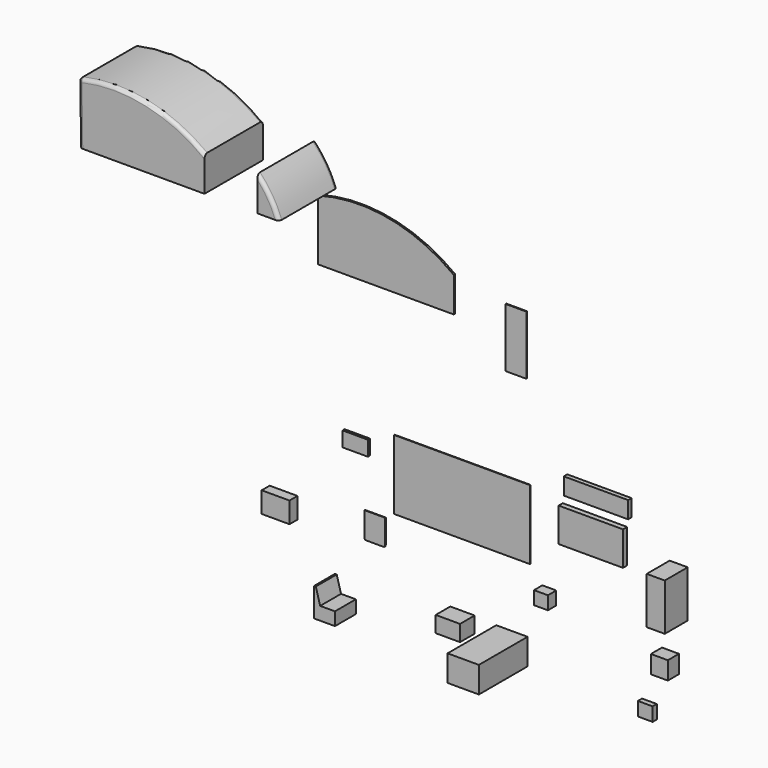
from build123d import *

# Parameters (mm, degrees)
F0_W      = 3962.4
F0_H      = 2032
F1_DEPTH  = 19.05
F0_W_2    = 527.05
F0_H_2    = 1371.6
F2_DEPTH  = 838.2
F0_W_3    = 495.3
F0_H_3    = 523.875
F3_DEPTH  = 406.4
F0_W_4    = 429.768
F0_H_4    = 400.05
F4_DEPTH  = 152.4
F0_W_5    = 741.68
F0_H_5    = 436.88
F5_DEPTH  = 76.2
F6_DEPTH  = 50.8
F7_DEPTH  = 19.05
F8_DEPTH  = 762
F9_DEPTH  = 2133.6
F0_W_6    = 609.6
F0_H_6    = 1727.2
F10_DEPTH = 25.4
F0_W_7    = 406.4
F0_H_7    = 387.35
F11_DEPTH = 304.8
F0_W_8    = 914.4
F0_H_8    = 762
F12_DEPTH = 1778
F0_W_9    = 711.2
F0_H_9    = 469.9
F13_DEPTH = 533.4
F14_DEPTH = 2133.6
F15_R     = 105.4762589975
F16_R     = 101.6
F16_2_R   = 101.6
F0_W_10   = 1879.6
F0_H_10   = 990.6
F17_DEPTH = 152.4
F18_DEPTH = 292.1
F0_H_11   = 495.3
F19_DEPTH = 127


# Not quite as in the source:
# - ends of sketch curves that miss each other by under 0.0002 mm in the source are joined


with BuildPart() as f1:
    # F0 (on Front) → F1 (new body)
    with BuildSketch(Plane.XZ):
        with Locations((-1277.7160794973, 1919.1620025635)):
            Rectangle(F0_W, F0_H)
    extrude(amount=F1_DEPTH)


with BuildPart() as f2:
    # F0 (on Front) → F2 (new body)
    with BuildSketch(Plane.XZ):
        with Locations((5036.8647483826, 1623.0339844704)):
            Rectangle(F0_W_2, F0_H_2)
    extrude(amount=F2_DEPTH)


with BuildPart() as f3:
    # F0 (on Front) → F3 (new body)
    with BuildSketch(Plane.XZ):
        with Locations((4797.2844566345, -261.9375)):
            Rectangle(F0_W_3, F0_H_3)
    extrude(amount=F3_DEPTH)


with BuildPart() as f4:
    # F0 (on Front) → F4 (new body)
    with BuildSketch(Plane.XZ):
        with Locations((4182.0682132568, -1700.6525627136)):
            Rectangle(F0_W_4, F0_H_4)
    extrude(amount=F4_DEPTH)


with BuildPart() as f5:
    # F0 (on Front) → F5 (new body)
    with BuildSketch(Plane.XZ):
        with Locations((-4351.5760449982, 2382.3956884766)):
            Rectangle(F0_W_5, F0_H_5)
    extrude(amount=F5_DEPTH)


with BuildPart() as f6:
    # F0 (on Front) → F6 (new body)
    with BuildSketch(Plane.XZ):
        with BuildLine():
            Line((-5455.5745124817, 8393.684387207), (-5455.5745124817, 6621.967618318))
            Line((-5455.5745124817, 6621.967618318), (-1493.1745124817, 6621.967618318))
            Line((-1493.1745124817, 6621.967618318), (-1493.1745124817, 7637.967618318))
            ThreePointArc((-1493.1745124817, 7637.967618318), (-3386.1147979663, 8478.5923554399), (-5455.5745124817, 8393.684387207))
        make_face()
    extrude(amount=F6_DEPTH)


with BuildPart() as f7:
    # F0 (on Front) → F7 (new body)
    with BuildSketch(Plane.XZ):
        with BuildLine():
            Line((-3521.931886673, 719.1577055931), (-4131.531886673, 719.1577055931))
            Line((-4131.531886673, 719.1577055931), (-4131.531886673, 7.9577055931))
            ThreePointArc((-4131.531886673, 7.9577055931), (-4116.6529111573, -27.9633188912), (-4080.731886673, -42.8422944069))
            Line((-4080.731886673, -42.8422944069), (-3572.731886673, -42.8422944069))
            ThreePointArc((-3572.731886673, -42.8422944069), (-3536.8108621887, -27.9633188912), (-3521.931886673, 7.9577055931))
            Line((-3521.931886673, 7.9577055931), (-3521.931886673, 719.1577055931))
        make_face()
    extrude(amount=F7_DEPTH)


with BuildPart() as f8:
    # F0 (on Front) → F8 (new body)
    with BuildSketch(Plane.XZ):
        Polygon((-4828.4018974304, -1668.460726738), (-4955.4018974304, -1211.260726738), (-5006.2018974304, -1211.260726738), (-5006.2018974304, -2049.460726738), (-4955.4018974304, -2049.460726738), (-4396.6018974304, -2049.460726738), (-4396.6018974304, -1668.460726738), align=None)
    extrude(amount=F8_DEPTH)


with BuildPart() as f9:
    # F0 (on Front) → F9 (new body)
    with BuildSketch(Plane.XZ):
        with BuildLine():
            Line((-10793.848991394, 10522.1261978149), (-10768.254913326, 8745.6674575806))
            Line((-10768.254913326, 8745.6674575806), (-7110.654913326, 8745.6674575806))
            Line((-7110.654913326, 8745.6674575806), (-7110.654913326, 9761.6674575806))
            ThreePointArc((-7110.654913326, 9761.6674575806), (-8866.9417812081, 10555.0867886532), (-10793.848991394, 10522.1261978149))
        make_face()
    extrude(amount=F9_DEPTH)

    # F15
    f15_edges = [f9.edges().sort_by_distance(p)[0] for p in [
        (-10793.848991, -1066.8, 10522.126198),
    ]]
    fillet(f15_edges, radius=F15_R)

    # F16
    f16_edges = [f9.edges().sort_by_distance(p)[0] for p in [
        (-10780.439396, -2133.6, 9591.379922),
        (-10780.439396, 0, 9591.379922),
    ]]
    fillet(f16_edges, radius=F16_R)


with BuildPart() as f10:
    # F0 (on Front) → F10 (new body)
    with BuildSketch(Plane.XZ):
        with Locations((304.8, 6504.5301757813)):
            Rectangle(F0_W_6, F0_H_6)
    extrude(amount=F10_DEPTH)


with BuildPart() as f11:
    # F0 (on Front) → F11 (new body)
    with BuildSketch(Plane.XZ):
        with Locations((1256.3688928604, 269.9453348637)):
            Rectangle(F0_W_7, F0_H_7)
    extrude(amount=F11_DEPTH)


with BuildPart() as f12:
    # F0 (on Front) → F12 (new body)
    with BuildSketch(Plane.XZ):
        with Locations((164.1450090408, -1381.5999803543)):
            Rectangle(F0_W_8, F0_H_8)
    extrude(amount=F12_DEPTH)


with BuildPart() as f13:
    # F0 (on Front) → F13 (new body)
    with BuildSketch(Plane.XZ):
        with Locations((-1280.7739883423, -1190.6021306038)):
            Rectangle(F0_W_9, F0_H_9)
    extrude(amount=F13_DEPTH)


with BuildPart() as f14:
    # F0 (on Front) → F14 (new body)
    with BuildSketch(Plane.XZ):
        with BuildLine():
            Line((-5568.809122225, 9761.6674575806), (-5568.809122225, 8745.6674575806))
            Line((-5568.809122225, 8745.6674575806), (-4931.2243461609, 8745.6674575806))
            ThreePointArc((-4931.2243461609, 8745.6674575806), (-5196.6883972792, 9287.1333392233), (-5568.809122225, 9761.6674575806))
        make_face()
    extrude(amount=F14_DEPTH)

    # F16#2
    f16_2_edges = [f14.edges().sort_by_distance(p)[0] for p in [
        (-5196.688397, -2133.6, 9287.133339),
        (-5196.688397, 0, 9287.133339),
    ]]
    fillet(f16_2_edges, radius=F16_2_R)


with BuildPart() as f17:
    # F0 (on Front) → F17 (new body)
    with BuildSketch(Plane.XZ):
        with Locations((2591.7781351089, 2275.894433403)):
            Rectangle(F0_W_10, F0_H_10)
    extrude(amount=F17_DEPTH)


with BuildPart() as f18:
    # F0 (on Front) → F18 (new body)
    with BuildSketch(Plane.XZ):
        Polygon((-6101.2024879456, -173.3167171478), (-6101.2024879456, 436.2832828522), (-6912.9147529602, 436.2832828522), (-6914.0024185181, -173.3167171478), align=None)
    extrude(amount=F18_DEPTH)


with BuildPart() as f19:
    # F0 (on Front) → F19 (new body)
    with BuildSketch(Plane.XZ):
        with Locations((2721.9534678528, 3307.1471179962)):
            Rectangle(F0_W_10, F0_H_11)
    extrude(amount=F19_DEPTH)


solid = Compound([f1.part, f2.part, f3.part, f4.part, f5.part, f6.part, f7.part, f8.part, f9.part, f10.part, f11.part, f12.part, f13.part, f14.part, f17.part, f18.part, f19.part])
